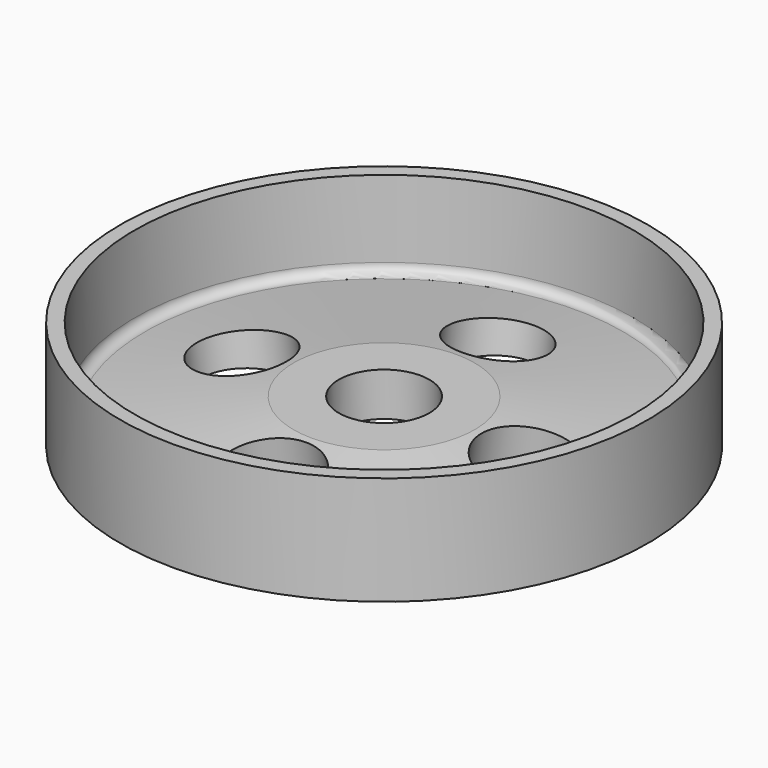
from build123d import *

# Parameters (mm, degrees)
F2_R            = 5
F3_DEPTH        = 4.8063913105
F5_R            = 5
F6_DEPTH        = 4.7469386033
F6_COPIES_COUNT = 4


# Not quite as in the source:
# - a pattern or mirror of a feature is missing from the dataset's text; its kind, count and spacing are read off the source's solid


with BuildPart() as f1:
    # F0 (on Right) → F1 (revolve)
    with BuildSketch(Plane.YZ):
        with BuildLine():
            Line((0, 0), (0, 4.8063913105))
            Line((0, 4.8063913105), (-10, 4.8063913105))
            Line((-10, 4.8063913105), (-26.410826899, 2.5))
            ThreePointArc((-26.410826899, 2.5), (-27.206059029, 2.7355584885), (-27.55, 3.4902680687))
            Line((-27.55, 3.4902680687), (-27.55, 12))
            Line((-27.55, 12), (-29.15, 12))
            Line((-29.15, 12), (-29.15, 0))
            Line((-29.15, 0), (0, 0))
        make_face()
    revolve(axis=Axis((0, 0, 11.0792994889), (0, 0, 1)))

    # F2 (on face) → F3 (cut, through all)
    with BuildSketch(Plane(origin=(0, 0, 0), x_dir=(1, 0, 0), z_dir=(0, 0, -1))):
        Circle(F2_R)
    extrude(amount=-F3_DEPTH, mode=Mode.SUBTRACT)

    # F5 (on line) → F6 (cut, through all)
    with BuildSketch(Plane(origin=(0, -0.8561020162, 6.0914823656), x_dir=(1, 0, 0), z_dir=(0, -0.139173101, 0.9902680687))):
        with Locations((0, -15)):
            Circle(F5_R)
    f6 = extrude(amount=-F6_DEPTH, mode=Mode.SUBTRACT)

    # F6_copies: F6 ×4 about axis
    f6_copies_axis = Axis((0, 0, 0), (0, 0, 1))
    for i in range(1, F6_COPIES_COUNT):
        add(f6.rotate(f6_copies_axis, i * 360 / F6_COPIES_COUNT), mode=Mode.SUBTRACT)


solid = f1.part
